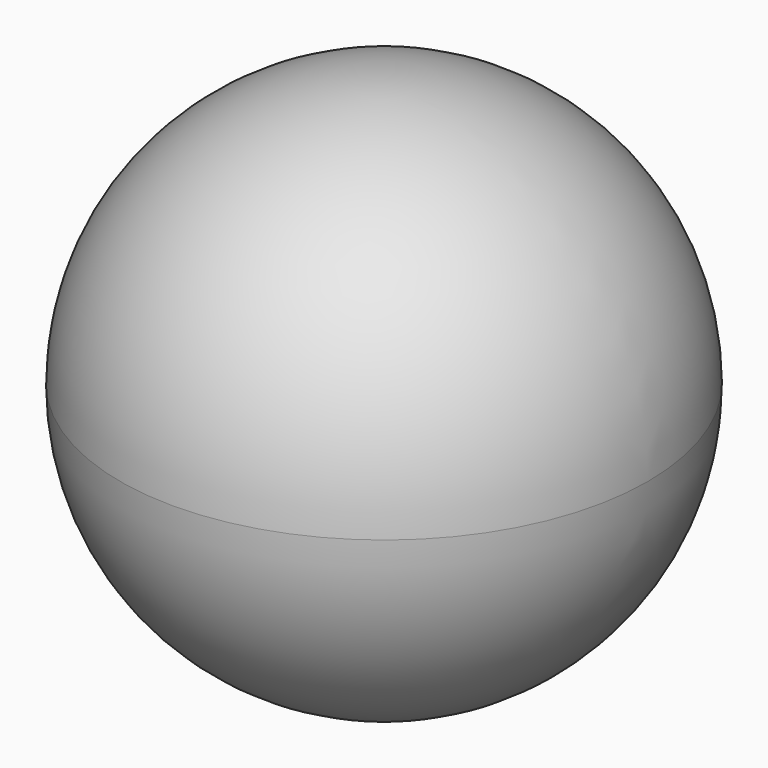
from build123d import *


with BuildPart() as f1:
    # F0 (on Front) → F1 (revolve)
    with BuildSketch(Plane.XZ):
        with BuildLine():
            ThreePointArc((0, -53.1687903206), (37.5960121832, -37.5960121832), (53.1687903206, 0))
            ThreePointArc((53.1687903206, 0), (37.5960121832, 37.5960121832), (0, 53.1687903206))
            Line((0, 53.1687903206), (0, 0))
            Line((0, 0), (0, -53.1687903206))
        make_face()
    revolve(axis=Axis((0, 0, 0), (0, 0, 1)))


solid = f1.part
